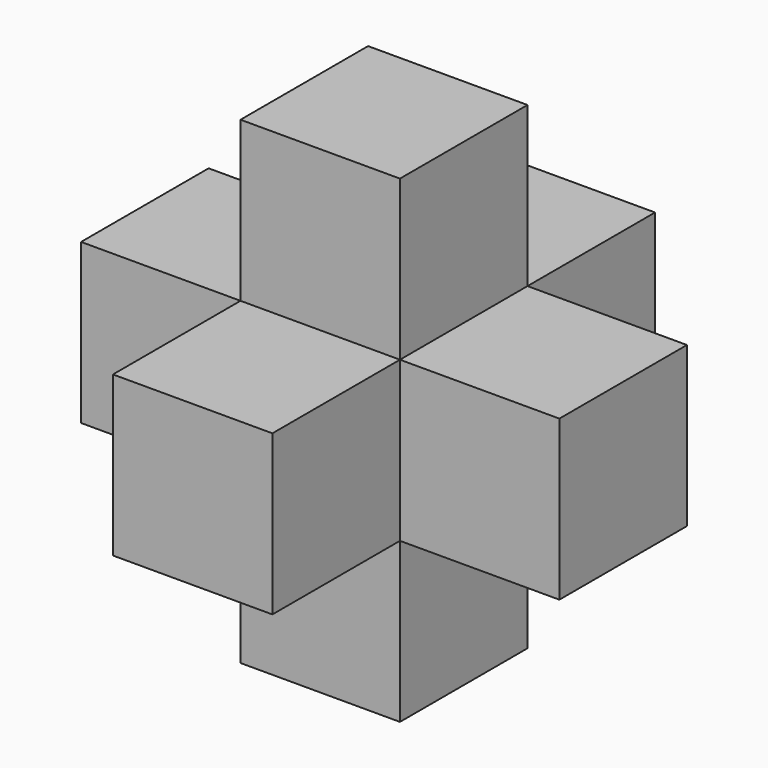
from build123d import *

# Parameters (mm, degrees)
F0_R      = 13.9889248678
F1_DEPTH  = 25.4
F2_SIZE   = 12.69999
F3_W      = 76.2
F3_H      = 76.2
F4_DEPTH  = 76.2
F5_W      = 25.4
F5_H      = 25.4
F7_DEPTH  = 76.2
F8_W      = 25.4
F8_H      = 25.4
F9_DEPTH  = 76.2
F10_W     = 25.4
F10_H     = 25.4
F11_DEPTH = 76.2


# Not quite as in the source:
# - a fillet or chamfer is up to 0.001 mm smaller than in the source, because OpenCascade refuses the exact size


with BuildPart() as f1:
    # F0 (on Top) → F1 (new body)
    with BuildSketch(Plane.XY):
        with Locations((-42.8192056715, -23.4777331352)):
            Circle(F0_R)
    extrude(amount=F1_DEPTH)

    # F2 (size 12.7 in the source; OpenCascade refuses exactly that, so slightly less here)
    f2_edges = [f1.edges().sort_by_distance(p)[0] for p in [
        (-28.830281, -23.477733, 12.7),
        (-56.808131, -23.477733, 0),
        (-56.808131, -23.477733, 25.4),
    ]]
    chamfer(f2_edges, length=F2_SIZE)


with BuildPart() as f4:
    # F3 (on Top) → F4 (new body)
    with BuildSketch(Plane.XY):
        with Locations((54.4739740274, 3.576669842)):
            Rectangle(F3_W, F3_H)
    extrude(amount=F4_DEPTH)

    # F5 (on face) → F7 (cut)
    with BuildSketch(Plane.XZ.offset(34.523330158)):
        with Locations((29.0739740274, 63.5)):
            Rectangle(F5_W, F5_H)
        with Locations((79.8739740274, 63.5)):
            Rectangle(F5_W, F5_H)
        with Locations((79.8739740274, 12.7)):
            Rectangle(F5_W, F5_H)
        with Locations((29.0739740274, 12.7)):
            Rectangle(F5_W, F5_H)
    extrude(amount=-F7_DEPTH, mode=Mode.SUBTRACT)

    # F8 (on face) → F9 (cut)
    with BuildSketch(Plane.YZ.offset(92.5739740274)):
        with Locations((-21.823330158, 12.7)):
            Rectangle(F8_W, F8_H)
        with Locations((-21.823330158, 63.5)):
            Rectangle(F8_W, F8_H)
        with Locations((28.976669842, 63.5)):
            Rectangle(F8_W, F8_H)
        with Locations((28.976669842, 12.7)):
            Rectangle(F8_W, F8_H)
    extrude(amount=-F9_DEPTH, mode=Mode.SUBTRACT)

    # F10 (on face) → F11 (cut)
    with BuildSketch(Plane.XY.offset(50.8)):
        with Locations((79.8739740274, -21.823330158)):
            Rectangle(F10_W, F10_H)
        with Locations((79.8739740274, 28.976669842)):
            Rectangle(F10_W, F10_H)
        with Locations((29.0739740274, 28.976669842)):
            Rectangle(F10_W, F10_H)
        with Locations((29.0739740274, -21.823330158)):
            Rectangle(F10_W, F10_H)
    extrude(amount=-F11_DEPTH, mode=Mode.SUBTRACT)


solid = f4.part
